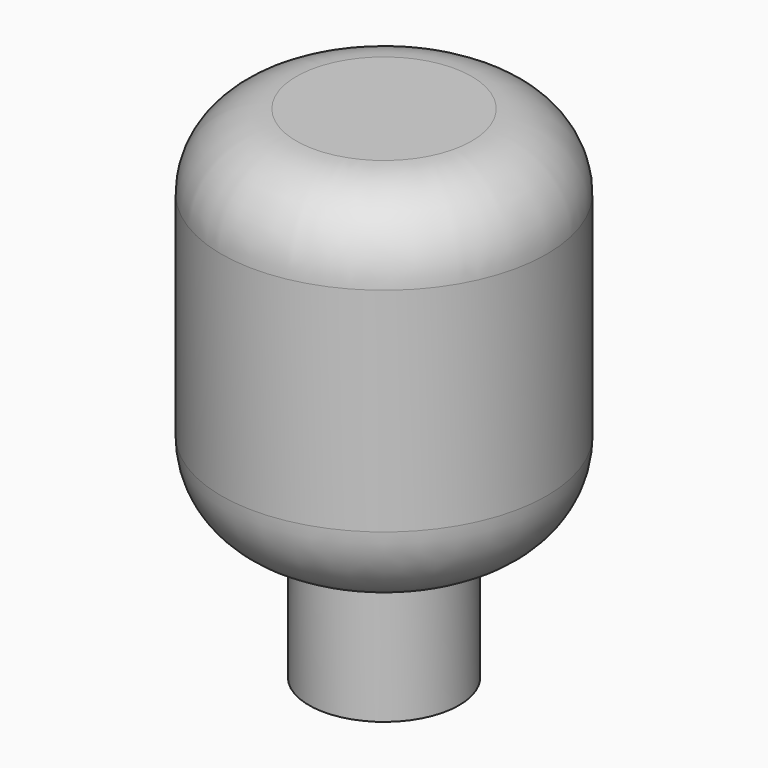
from build123d import *

# Parameters (mm, degrees)
F0_R     = 6.5
F1_DEPTH = 15
F2_R     = 3
F2_R_2   = 1.5
F3_DEPTH = 5
F4_R     = 3.49999
F5_R     = 3


# Not quite as in the source:
# - a fillet or chamfer is up to 0.001 mm smaller than in the source, because OpenCascade refuses the exact size


with BuildPart() as f1:
    # F0 (on Top) → F1 (new body)
    with BuildSketch(Plane.XY):
        Circle(F0_R)
    extrude(amount=F1_DEPTH)

    # F2 (on face) → F3 (join)
    with BuildSketch(Plane(origin=(0, 0, 0), x_dir=(1, 0, 0), z_dir=(0, 0, -1))):
        Circle(F2_R)
        Circle(F2_R_2, mode=Mode.SUBTRACT)
    extrude(amount=F3_DEPTH)

    # F4 (radius 3.5 in the source; OpenCascade refuses exactly that, so slightly less here)
    f4_edges = [f1.edges().sort_by_distance(p)[0] for p in [
        (-6.5, 0, 0),
    ]]
    fillet(f4_edges, radius=F4_R)

    # F5
    f5_edges = [f1.edges().sort_by_distance(p)[0] for p in [
        (-6.5, 0, 15),
    ]]
    fillet(f5_edges, radius=F5_R)


solid = f1.part
